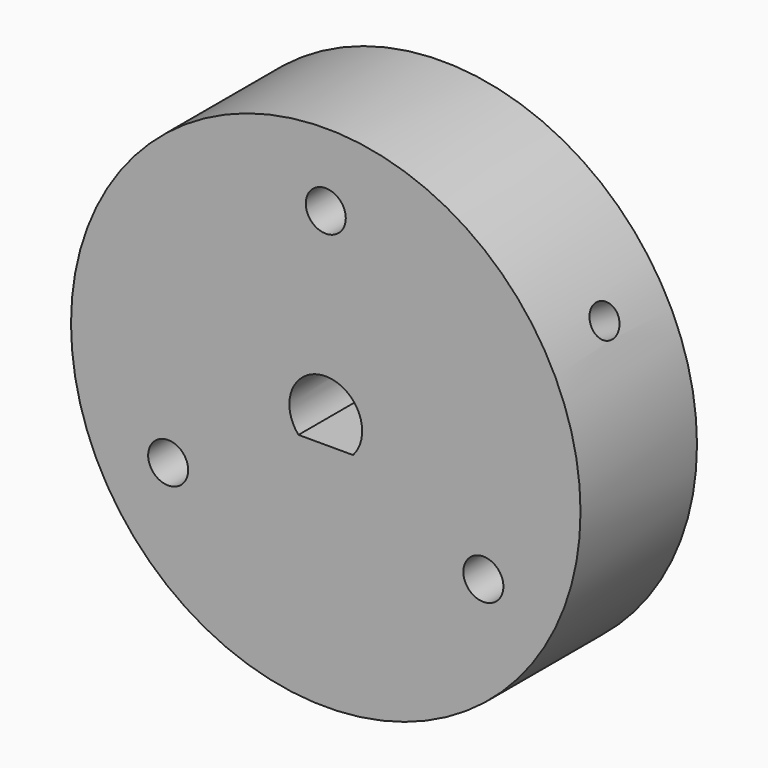
from build123d import *

# Parameters (mm, degrees)
F0_R     = 14
F0_R_2   = 1.1
F1_DEPTH = 8
F3_DEPTH = 8.001
F6_R     = 0.875
F7_DEPTH = 19.125355653


# Not quite as in the source:
# - a pattern or mirror of a feature is missing from the dataset's text; its kind, count and spacing are read off the source's solid


with BuildPart() as f1:
    # F0 (on Front) → F1 (new body)
    with BuildSketch(Plane.XZ):
        Circle(F0_R)
        with Locations((-8.6602540378, -5)):
            Circle(F0_R_2, mode=Mode.SUBTRACT)
        with Locations((8.6602540378, -5)):
            Circle(F0_R_2, mode=Mode.SUBTRACT)
        with Locations((0, 10)):
            Circle(F0_R_2, mode=Mode.SUBTRACT)
    extrude(amount=F1_DEPTH)

    # F2 (on face) → F3 (cut, through all)
    with BuildSketch(Plane.XZ.offset(8)):
        with BuildLine():
            Line((-1.5, -1.3228756555), (1.5, -1.3228756555))
            ThreePointArc((1.5, -1.3228756555), (0, 2), (-1.5, -1.3228756555))
        make_face()
    extrude(amount=-F3_DEPTH, mode=Mode.SUBTRACT)

    # F6 (on line) → F7 (cut, through all)
    with BuildSketch(Plane(origin=(0, 0, 0), x_dir=(0, 1, 0), z_dir=(0.8660254038, 0, -0.5))):
        with Locations((-4, 0)):
            Circle(F6_R)
    f7 = extrude(amount=-F7_DEPTH, mode=Mode.SUBTRACT)

    # F7_copies: F7 across plane
    add(f7.mirror(Plane(origin=(1.9e-05, 0, 0), x_dir=(-1e-06, 0, 1), z_dir=(1, 0, 1e-06))), mode=Mode.SUBTRACT)


solid = f1.part
